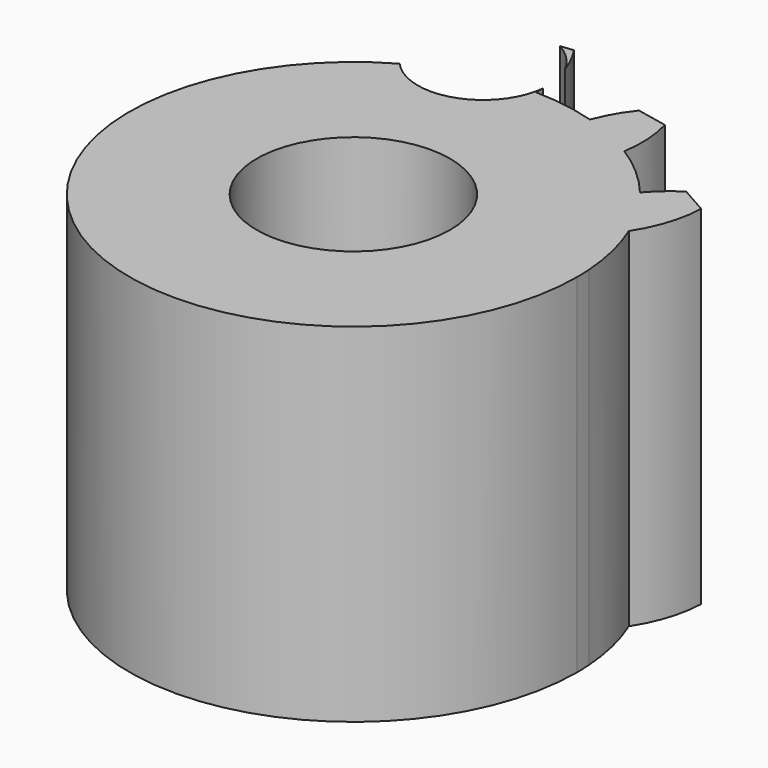
from build123d import *

# Parameters (mm, degrees)
F2_R     = 2
F3_DEPTH = 7.2


# Not quite as in the source:
# - a feature of the source that left no trace in its solid (it failed there, or was rolled back) is left out


with BuildPart() as f3:
    # F2 (on Top) → F3 (new body)
    with BuildSketch(Plane.XY):
        with BuildLine():
            ThreePointArc((-2.271785382, 4.0357734997), (-2.3374420327, -3.9981047143), (4.63125, 0))
            ThreePointArc((4.63125, 0), (4.6285496159, 0.1581297427), (4.6204516127, 0.3160750811))
            ThreePointArc((4.6204516127, 0.3160750811), (4.5082656604, 1.0601968205), (4.2770482379, 1.7763262462))
            ThreePointArc((4.2770482379, 1.7763262462), (3.9694318812, 2.3858095278), (3.5755556432, 2.943446688))
            ThreePointArc((3.5755556432, 2.943446688), (3.0649914702, 3.4719308533), (2.4772652952, 3.9130082059))
            ThreePointArc((2.4772652952, 3.9130082059), (1.9312745013, 4.2093533189), (1.3505339311, 4.4299587654))
            ThreePointArc((1.3505339311, 4.4299587654), (0.7199844888, 4.5749425022), (0.0753830097, 4.6306364535))
            ThreePointArc((0.0753830097, 4.6306364535), (0.0603841431, 4.6308563266), (0.0453846431, 4.6310276178))
            ThreePointArc((0.0453846431, 4.6310276178), (-0.9332314655, 3.6328282536), (-2.271785382, 4.0357734997))
        make_face()
        Circle(F2_R, mode=Mode.SUBTRACT)
        with BuildLine():
            ThreePointArc((3.5755556432, 2.943446688), (3.9694318812, 2.3858095278), (4.2770482379, 1.7763262462))
            ThreePointArc((4.2770482379, 1.7763262462), (4.5827309803, 2.4158772636), (4.7053196857, 3.1140459053))
            Line((4.7053196857, 3.1140459053), (4.1375685599, 3.436199056))
            ThreePointArc((4.1375685599, 3.436199056), (3.8388567011, 3.2100169175), (3.5755556432, 2.943446688))
        make_face()
        with BuildLine():
            ThreePointArc((0.0747314467, 4.8064535177), (0.0629485737, 4.7182570144), (0.0453846431, 4.6310276178))
            ThreePointArc((0.0453846431, 4.6310276178), (0.0603841431, 4.6308563266), (0.0753830097, 4.6306364535))
            ThreePointArc((0.0753830097, 4.6306364535), (0.0765360395, 4.7185504659), (0.0747314467, 4.8064535177))
        make_face()
        with BuildLine():
            ThreePointArc((1.3505339311, 4.4299587654), (1.9312745013, 4.2093533189), (2.4772652952, 3.9130082059))
            ThreePointArc((2.4772652952, 3.9130082059), (2.5058690535, 4.4804717295), (2.411165728, 5.0407076671))
            Line((2.411165728, 5.0407076671), (1.7716515219, 5.1716487739))
            ThreePointArc((1.7716515219, 5.1716487739), (1.5306343406, 4.8180974664), (1.3505339311, 4.4299587654))
        make_face()
    extrude(amount=F3_DEPTH)


with BuildPart() as f3b:
    # F2 (on Top) → F3, piece 2 (new body)
    with BuildSketch(Plane.XY):
        with BuildLine():
            Line((-0.3660755696, 6.1641393298), (-0.6351975831, 6.1338165614))
            ThreePointArc((-0.6351975831, 6.1338165614), (-0.3016496515, 5.883587861), (-0.0603117652, 5.5435516133))
            ThreePointArc((-0.0603117652, 5.5435516133), (-0.1925694184, 5.8640070469), (-0.3660755696, 6.1641393298))
        make_face()
    extrude(amount=F3_DEPTH)


solid = Compound([f3.part, f3b.part])
